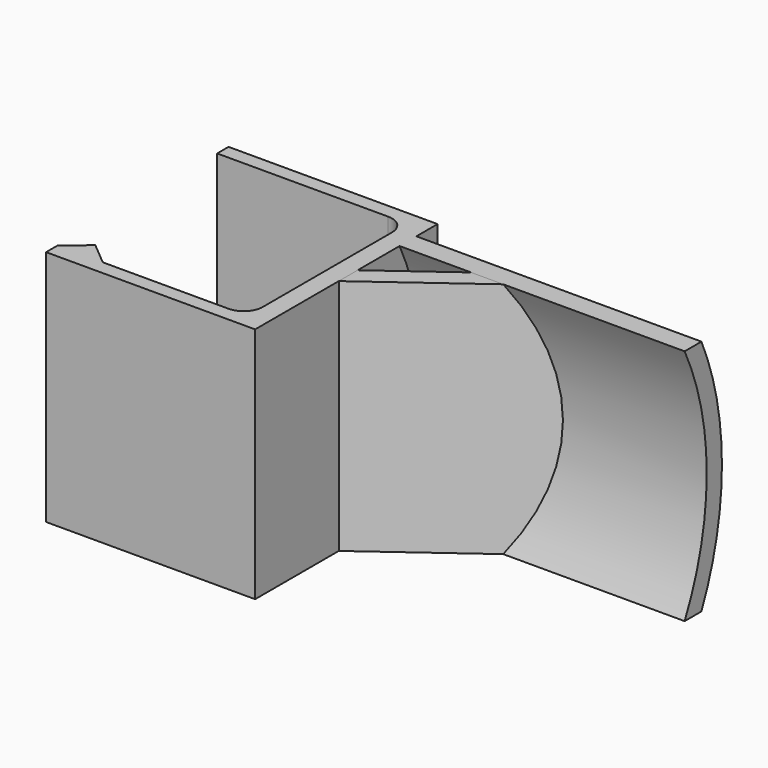
from build123d import *

# Parameters (mm, degrees)
F1_DEPTH    = 25
F3_DEPTH    = 30
F4_DEPTH    = 25
F5_T1_DEPTH = 18.3820136796


# Not quite as in the source:
# - a fillet or chamfer that OpenCascade refuses, or shapes differently, is made with other operations: its cross-section is extruded or revolved along the edge and cut away or added


with BuildPart() as f1:
    # F0 (on Top) → F1 (new body)
    with BuildSketch(Plane.XY):
        with BuildLine():
            Line((0, 22.5), (-22, 22.5))
            Line((-22, 22.5), (-22, 21))
            Line((-22, 21), (-17.2329856296, 21))
            Line((-17.2329856296, 21), (-4, 21))
            ThreePointArc((-4, 21), (-2.5857864376, 20.4142135624), (-2, 19))
            Line((-2, 19), (-2, 10.5))
            Line((-2, 10.5), (-2, 2))
            ThreePointArc((-2, 2), (-2.5857864376, 0.5857864376), (-4, 0))
            Line((-4, 0), (-17.2329856296, 0))
            Line((-17.2329856296, 0), (-22, 0))
            Line((-22, 0), (-22, -1.5))
            Line((-22, -1.5), (-2, -1.5))
            Line((-2, -1.5), (0, -1.5))
            Line((0, -1.5), (0, 9.5))
            Line((0, 9.5), (0, 11.980143365))
            Line((0, 11.980143365), (0, 17.5))
            Line((0, 17.5), (0, 22.5))
        make_face()
        Polygon((-19.6164928148, 2), (-22, 0), (-17.2329856296, 0), align=None)
    extrude(amount=F1_DEPTH)

    # F2 (on face) → F3 (join)
    with BuildSketch(Plane.YZ):
        with BuildLine():
            ThreePointArc((17.5, 25), (20.40460778, 12.5), (17.5, 0))
            Line((17.5, 0), (19.7108604723, 0))
            ThreePointArc((19.7108604723, 0), (22.40460778, 12.5), (19.7108604723, 25))
            Line((19.7108604723, 25), (17.5, 25))
        make_face()
    extrude(amount=F3_DEPTH)


with BuildPart() as f4:
    # F0 (on Top) → F4 (new body)
    with BuildSketch(Plane.XY):
        Polygon((11.6179863204, 20.5), (0, 11.980143365), (0, 9.5), (15, 20.5), align=None)
    extrude(amount=F4_DEPTH)

    # F5: fillet of radius 3 on 2 edges, made by hand

    # F5_s2 → F5_t1 (cut)
    with BuildSketch(Plane.YZ.offset(4.1179863204)):
        with BuildLine():
            ThreePointArc((20.5, 22), (19.6213203436, 24.1213203436), (17.5, 25))
            Line((17.5, 25), (20.5, 25))
            Line((20.5, 25), (20.5, 22))
        make_face()
        with BuildLine():
            ThreePointArc((20.5, 3), (19.6213203436, 0.8786796564), (17.5, 0))
            Line((17.5, 0), (20.5, 0))
            Line((20.5, 0), (20.5, 3))
        make_face()
    extrude(amount=F5_T1_DEPTH, mode=Mode.SUBTRACT)


solid = Compound([f1.part, f4.part])
